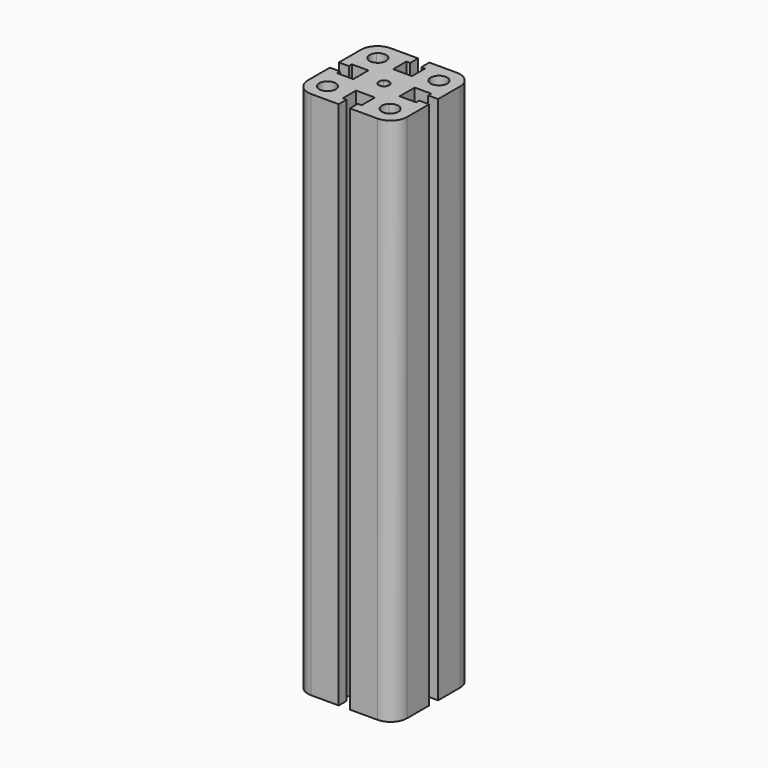
from build123d import *

# Parameters (mm, degrees)
F0_W     = 1.15
F0_H     = 3
F0_W_2   = 3
F0_H_2   = 1.15
F1_DEPTH = 160
F2_R     = 5
F4_DEPTH = 200


with BuildPart() as f1:
    # F0 (on Top) → F1 (new body)
    with BuildSketch(Plane.XY):
        with BuildLine():
            Line((7.5, 7.5), (15, 15))
            Line((15, 15), (2.85, 15))
            Line((2.85, 15), (2.85, 12))
            Line((2.85, 12), (2.85, 7))
            Line((2.85, 7), (0, 7))
            Line((0, 7), (0, 1.55))
            ThreePointArc((0, 1.55), (0.5931593202, 1.4320132754), (1.0960155108, 1.0960155108))
            Line((1.0960155108, 1.0960155108), (7.5, 7.5))
        make_face()
        with BuildLine():
            Line((15, 2.85), (15, 15))
            Line((15, 15), (7.5, 7.5))
            Line((7.5, 7.5), (1.0960155108, 1.0960155108))
            ThreePointArc((1.0960155108, 1.0960155108), (1.4320132754, 0.5931593202), (1.55, 0))
            ThreePointArc((1.55, 0), (1.4320132754, -0.5931593202), (1.0960155108, -1.0960155108))
            Line((1.0960155108, -1.0960155108), (7.5, -7.5))
            Line((7.5, -7.5), (15, -15))
            Line((15, -15), (15, -2.85))
            Line((15, -2.85), (12, -2.85))
            Line((12, -2.85), (7, -2.85))
            Line((7, -2.85), (7, 2.85))
            Line((7, 2.85), (12, 2.85))
            Line((12, 2.85), (15, 2.85))
        make_face()
        with Locations((2.275, 13.5)):
            Rectangle(F0_W, F0_H)
        with Locations((13.5, 2.275)):
            Rectangle(F0_W_2, F0_H_2)
        with BuildLine():
            ThreePointArc((-1.0960155108, 1.0960155108), (-0.5931593202, 1.4320132754), (0, 1.55))
            Line((0, 1.55), (0, 7))
            Line((0, 7), (-2.85, 7))
            Line((-2.85, 7), (-2.85, 12))
            Line((-2.85, 12), (-2.85, 15))
            Line((-2.85, 15), (-15, 15))
            Line((-15, 15), (-7.5, 7.5))
            Line((-7.5, 7.5), (-1.0960155108, 1.0960155108))
        make_face()
        with Locations((-2.275, 13.5)):
            Rectangle(F0_W, F0_H)
        with Locations((13.5, -2.275)):
            Rectangle(F0_W_2, F0_H_2)
        with BuildLine():
            Line((7.5, -7.5), (1.0960155108, -1.0960155108))
            ThreePointArc((1.0960155108, -1.0960155108), (0, -1.55), (-1.0960155108, -1.0960155108))
            Line((-1.0960155108, -1.0960155108), (-7.5, -7.5))
            Line((-7.5, -7.5), (-15, -15))
            Line((-15, -15), (-2.85, -15))
            Line((-2.85, -15), (-2.85, -12))
            Line((-2.85, -12), (-2.85, -7))
            Line((-2.85, -7), (2.85, -7))
            Line((2.85, -7), (2.85, -12))
            Line((2.85, -12), (2.85, -15))
            Line((2.85, -15), (15, -15))
            Line((15, -15), (7.5, -7.5))
        make_face()
        with BuildLine():
            ThreePointArc((-1.0960155108, -1.0960155108), (-1.55, 0), (-1.0960155108, 1.0960155108))
            Line((-1.0960155108, 1.0960155108), (-7.5, 7.5))
            Line((-7.5, 7.5), (-15, 15))
            Line((-15, 15), (-15, 2.85))
            Line((-15, 2.85), (-12, 2.85))
            Line((-12, 2.85), (-7, 2.85))
            Line((-7, 2.85), (-7, -2.85))
            Line((-7, -2.85), (-12, -2.85))
            Line((-12, -2.85), (-15, -2.85))
            Line((-15, -2.85), (-15, -15))
            Line((-15, -15), (-7.5, -7.5))
            Line((-7.5, -7.5), (-1.0960155108, -1.0960155108))
        make_face()
        with Locations((-13.5, 2.275)):
            Rectangle(F0_W_2, F0_H_2)
        with Locations((2.275, -13.5)):
            Rectangle(F0_W, F0_H)
        with Locations((-2.275, -13.5)):
            Rectangle(F0_W, F0_H)
        with Locations((-13.5, -2.275)):
            Rectangle(F0_W_2, F0_H_2)
    extrude(amount=F1_DEPTH)

    # F2
    f2_edges = [f1.edges().sort_by_distance(p)[0] for p in [
        (15, -15, 80),
        (-15, -15, 80),
        (15, 15, 80),
        (-15, 15, 80),
    ]]
    fillet(f2_edges, radius=F2_R)

    # F3 (on face) → F4 (cut)
    with BuildSketch(Plane.XY.offset(160)):
        with BuildLine():
            ThreePointArc((-7, -9.5), (-7.1903011687, -8.5432914191), (-7.732233047, -7.732233047))
            Line((-7.732233047, -7.732233047), (-11.267766953, -11.267766953))
            ThreePointArc((-11.267766953, -11.267766953), (-8.5432914191, -11.8096988313), (-7, -9.5))
        make_face()
        with BuildLine():
            Line((-11.267766953, -11.267766953), (-7.732233047, -7.732233047))
            ThreePointArc((-7.732233047, -7.732233047), (-11.267766953, -7.732233047), (-11.267766953, -11.267766953))
        make_face()
        with BuildLine():
            ThreePointArc((11.730266953, -9.230266953), (10.1869755339, -6.9205681217), (7.4625, -7.4625))
            Line((7.4625, -7.4625), (10.9980339059, -10.9980339059))
            ThreePointArc((10.9980339059, -10.9980339059), (11.5399657842, -10.1869755339), (11.730266953, -9.230266953))
        make_face()
        with BuildLine():
            Line((10.9980339059, -10.9980339059), (7.4625, -7.4625))
            ThreePointArc((7.4625, -7.4625), (7.4625, -10.9980339059), (10.9980339059, -10.9980339059))
        make_face()
        with BuildLine():
            ThreePointArc((10.9980339059, 10.9980339059), (7.4625, 10.9980339059), (7.4625, 7.4625))
            Line((7.4625, 7.4625), (10.9980339059, 10.9980339059))
        make_face()
        with BuildLine():
            Line((10.9980339059, 10.9980339059), (7.4625, 7.4625))
            ThreePointArc((7.4625, 7.4625), (10.1869755339, 6.9205681217), (11.730266953, 9.230266953))
            ThreePointArc((11.730266953, 9.230266953), (11.5399657842, 10.1869755339), (10.9980339059, 10.9980339059))
        make_face()
        with BuildLine():
            ThreePointArc((-10.9980339059, 10.9980339059), (-10.9980339059, 7.4625), (-7.4625, 7.4625))
            Line((-7.4625, 7.4625), (-10.9980339059, 10.9980339059))
        make_face()
        with BuildLine():
            Line((-10.9980339059, 10.9980339059), (-7.4625, 7.4625))
            ThreePointArc((-7.4625, 7.4625), (-6.9205681217, 8.2735583721), (-6.730266953, 9.230266953))
            ThreePointArc((-6.730266953, 9.230266953), (-8.2735583721, 11.5399657842), (-10.9980339059, 10.9980339059))
        make_face()
    extrude(amount=-F4_DEPTH, mode=Mode.SUBTRACT)


solid = f1.part
